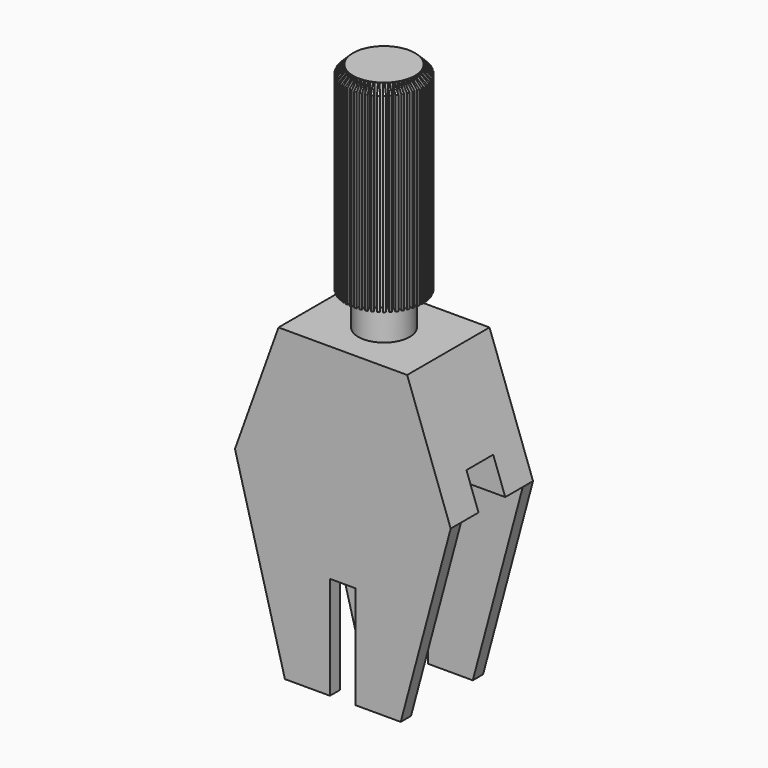
from build123d import *

# Parameters (mm, degrees)
F1_DEPTH         = 200
F4_DEPTH         = 500
F7_R             = 65
F7_R_2           = 50
F8_DEPTH         = 100
F9_DEPTH         = 350
F11_DEPTH        = 65
F12_SIZE         = 30
F13_W            = 42.0357882977
F13_H            = 10
F14_DEPTH        = 770
F14_COPIES_COUNT = 50


# Not quite as in the source:
# - a pattern or mirror of a feature is missing from the dataset's text; its kind, count and spacing are read off the source's solid


with BuildPart() as f1:
    # F0 (on Front) → F1 (new body, symmetric)
    with BuildSketch(Plane.XZ):
        Polygon((-50, 180.4053897521), (0, 180.4053897521), (0, 975.381755199), (-250, 975.381755199), (-419.1142838269, 504.8497594689), (-225, -219.5946102479), (-50, -219.5946102479), align=None)
    extrude(amount=F1_DEPTH, both=True)

    # F2: F1 across plane


with BuildPart() as f1_1:
    add(f1.part)
    add(f1.part.mirror(Plane.YZ))

    # F3 (on Right) → F4 (cut, symmetric)
    with BuildSketch(Plane.YZ):
        Polygon((-150, 504.8497594689), (-150, -219.5946102479), (150, -219.5946102479), (150, 504.8497594689), (65, 504.8497594689), (65, 634.8497594689), (-65, 634.8497594689), (-65, 504.8497594689), align=None)
    extrude(amount=F4_DEPTH, both=True, mode=Mode.SUBTRACT)

    # F5 (on Front) → F6 (revolve)
    with BuildSketch(Plane.XZ):
        Polygon((-100, 1105.381755199), (-100, 975.381755199), (0, 975.381755199), (0, 1875.381755199), (-150, 1875.381755199), (-150, 1105.381755199), align=None)
    revolve(axis=Axis((0, 0, 1425.381755199), (0, 0, 1)))

    # F7 (on face) → F8 (cut)
    with BuildSketch(Plane(origin=(0, 200, 0), x_dir=(-1, 0, 0), z_dir=(0, 1, 0))):
        with Locations((-129.1142838269, 645.381755199)):
            Circle(F7_R)
        with Locations((-129.1142838269, 645.381755199)):
            Circle(F7_R_2, mode=Mode.SUBTRACT)
    f8 = extrude(amount=-F8_DEPTH, mode=Mode.SUBTRACT)

    # F8_copies: F8 across plane
    add(f8.mirror(Plane(origin=(0, 0, 0), x_dir=(0, 0, -1), z_dir=(-1, 0, 0))), mode=Mode.SUBTRACT)

    # F9 (cut): a face of the model
    f9_faces = [f1_1.faces().sort_by_distance(p)[0] for p in [
        (129.1142838269, 200, 645.381755199),
    ]]
    f9 = extrude(f9_faces, amount=-F9_DEPTH, mode=Mode.SUBTRACT)

    # F9_copies: F9 across plane
    add(f9.mirror(Plane(origin=(0, 0, 0), x_dir=(0, 0, -1), z_dir=(-1, 0, 0))), mode=Mode.SUBTRACT)

    # F10 (on Front) → F11 (cut, symmetric)
    with BuildSketch(Plane.XZ):
        Polygon((-419.1142838269, 504.8497594689), (419.1142838269, 504.8497594689), (372.3908790489, 634.8497594689), (293.9095679375, 705.381755199), (268.7508115185, 775.381755199), (-268.7508115185, 775.381755199), (-293.9095679375, 705.381755199), (-372.3908790489, 634.8497594689), align=None)
    extrude(amount=F11_DEPTH, both=True, mode=Mode.SUBTRACT)

    # F12
    f12_edges = [f1_1.edges().sort_by_distance(p)[0] for p in [
        (150, 0, 1875.381755),
    ]]
    chamfer(f12_edges, length=F12_SIZE)

    # F13 (on face) → F14 (cut)
    with BuildSketch(Plane.XY.offset(1875.381755199)):
        with Locations((141.0178941488, -10.0858946145)):
            Rectangle(F13_W, F13_H)
    f14 = extrude(amount=-F14_DEPTH, mode=Mode.SUBTRACT)

    # F14_copies: F14 ×50 about axis
    f14_copies_axis = Axis((0, 0, 0), (0, 0, 1))
    for i in range(1, F14_COPIES_COUNT):
        add(f14.rotate(f14_copies_axis, i * 360 / F14_COPIES_COUNT), mode=Mode.SUBTRACT)


solid = f1_1.part
